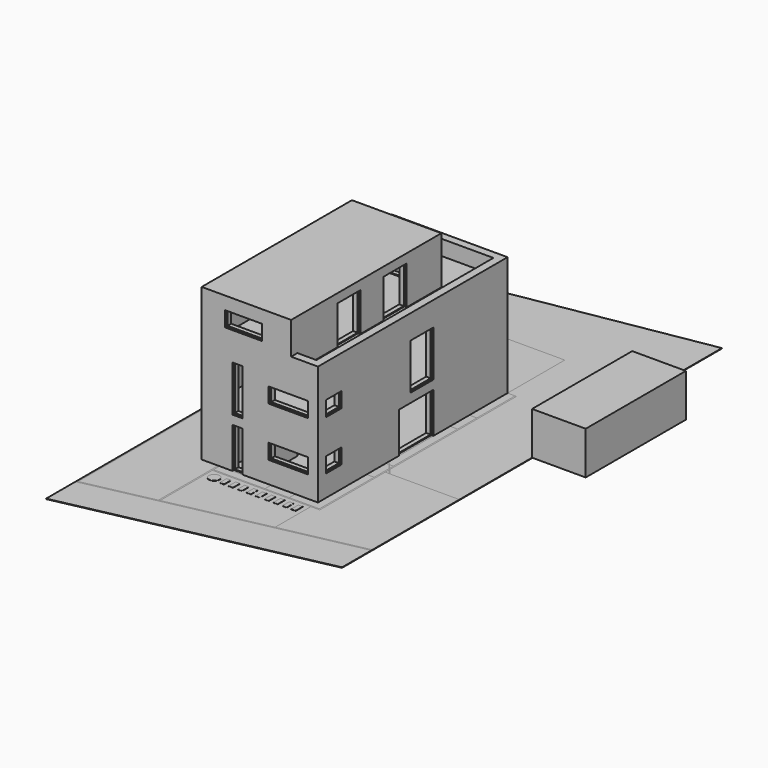
from build123d import *

# Parameters (mm, degrees)
F0_W      = 6500
F0_H      = 13250
F2_DEPTH  = 25
F3_DEPTH  = 2270
F1_W      = 150
F1_H      = 3500
F5_W      = 365
F5_H      = 1100
F5_W_2    = 2200
F5_H_2    = 365
F5_H_3    = 500
F6_DEPTH  = 850
F7_W      = 6500
F7_H      = 13250
F7_W_2    = 990
F7_H_2    = 2385
F8_DEPTH  = 300
F9_W      = 150
F9_H      = 3500
F10_DEPTH = 300
F11_W     = 6500
F11_H     = 13250
F12_DEPTH = 200
F14_DEPTH = 2570
F16_W     = 2200
F16_H     = 365
F16_W_2   = 365
F16_H_2   = 1100
F17_DEPTH = 850
F18_W     = 6500
F18_H     = 13250
F18_W_2   = 5770
F18_H_2   = 12520
F19_DEPTH = 300
F21_W     = 2400
F21_H     = 365
F22_DEPTH = 1280
F23_W     = 6500
F23_H     = 13250
F24_DEPTH = 200
F25_W     = 365
F25_H     = 1630
F26_DEPTH = 2160
F28_W     = 2050
F28_H     = 365
F29_DEPTH = 850
F30_W     = 5000
F30_H     = 10500
F30_W_2   = 4270
F30_H_2   = 9770
F31_DEPTH = 300
F32_W     = 5000
F32_H     = 10500
F33_DEPTH = 200
F35_DEPTH = 850
F38_DEPTH = 2200
F39_W     = 3000
F39_H     = 6000
F40_DEPTH = 25
F41_W     = 3000
F41_H     = 6000
F42_DEPTH = 200
F44_DEPTH = 25
F46_DEPTH = 25
F47_W     = 2880
F47_H     = 420
F48_DEPTH = 25
F47_W_2   = 420
F47_H_2   = 2670
F47_H_3   = 4480
F50_DEPTH = 25
F51_W     = 1350
F51_H     = 420
F52_DEPTH = 25
F51_W_2   = 420
F51_H_2   = 1350
F54_DEPTH = 25
F56_DEPTH = 25
F58_DEPTH = 25
F60_DEPTH = 25
F61_W     = 3000
F61_H     = 7000
F62_DEPTH = 2400
F63_R     = 1525
F64_DEPTH = 200
F65_R     = 1525
F65_R_2   = 1515
F66_DEPTH = 1800
F68_DEPTH = 25
F69_R     = 300
F70_DEPTH = 10
F71_W     = 250
F71_H     = 500
F72_DEPTH = 10
F74_DEPTH = 25
F76_DEPTH = 25
F77_W     = 570
F77_H     = 2570
F77_W_2   = 470
F77_H_2   = 2470
F78_DEPTH = 250
F77_W_3   = 2200
F77_H_3   = 850
F77_W_4   = 2100
F77_H_4   = 750
F77_W_5   = 2050
F77_W_6   = 1950
F77_H_5   = 2270
F77_H_6   = 2170
F79_W     = 2400
F79_H     = 2270
F79_W_2   = 2300
F79_H_2   = 2170
F80_DEPTH = 250
F79_W_3   = 1100
F79_H_3   = 850
F79_W_4   = 1000
F79_H_4   = 750
F79_W_5   = 1600
F79_H_5   = 2570
F79_W_6   = 1500
F79_H_6   = 2470
F81_W     = 1600
F81_H     = 2160
F81_W_2   = 1500
F81_H_2   = 2060
F82_DEPTH = 250
F83_W     = 2400
F83_H     = 1280
F83_W_2   = 2300
F83_H_2   = 1180
F84_DEPTH = 250
F83_H_3   = 2270
F83_H_4   = 2170
F85_W     = 2400
F85_H     = 2160
F85_W_2   = 2300
F85_H_2   = 2060
F86_DEPTH = 250
F87_W     = 570
F87_H     = 2570
F87_W_2   = 470
F87_H_2   = 2470
F88_DEPTH = 250
F87_W_3   = 1100
F87_H_3   = 2270
F87_W_4   = 1000
F87_H_4   = 2170
F87_W_5   = 500
F87_H_5   = 850
F87_W_6   = 400
F87_H_6   = 750
F89_W     = 2700
F89_H     = 2200
F90_DEPTH = 25
F91_W     = 850
F91_H     = 2200
F92_DEPTH = 25


with BuildPart() as f2:
    # F0 (on Top) → F2 (new body)
    with BuildSketch(Plane.XY):
        with Locations((3250, 6625)):
            Rectangle(F0_W, F0_H)
    extrude(amount=-F2_DEPTH)


with BuildPart() as f3:
    # F1 (on Top) → F3 (new body)
    with BuildSketch(Plane.XY):
        Polygon((2050, 12885), (2050, 13250), (0, 13250), (0, 4000), (365, 4000), (365, 12885), align=None)
    extrude(amount=F3_DEPTH)



with BuildPart() as f3b:
    # F1 (on Top) → F3, piece 2 (new body)
    with BuildSketch(Plane.XY):
        Polygon((4450, 13250), (4450, 12885), (6135, 12885), (6135, 8065), (6500, 8065), (6500, 13250), align=None)
    extrude(amount=F3_DEPTH)


with BuildPart() as f3c:
    # F1 (on Top) → F3, piece 3 (new body)
    with BuildSketch(Plane.XY):
        Polygon((6500, 5665), (6135, 5665), (6135, 1655), (6135, 555), (6135, 365), (5945, 365), (3745, 365), (3055, 365), (2955, 365), (2280, 365), (2280, 0), (3745, 0), (5945, 0), (6500, 0), (6500, 555), (6500, 1655), align=None)
        Polygon((2955, 365), (3055, 365), (3055, 2860), (2455, 2860), (2455, 2760), (2955, 2760), align=None)
    extrude(amount=F3_DEPTH)


with BuildPart() as f3d:
    # F1 (on Top) → F3, piece 4 (new body)
    with BuildSketch(Plane.XY):
        Polygon((1710, 0), (1710, 365), (1455, 365), (1355, 365), (365, 365), (365, 1400), (365, 1900), (365, 2750), (365, 2900), (0, 2900), (0, 1900), (0, 1400), (0, 0), align=None)
        Polygon((1355, 365), (1455, 365), (1455, 2900), (365, 2900), (365, 2750), (1355, 2750), align=None)
    extrude(amount=F3_DEPTH)


with BuildPart() as f3e:
    # F1 (on Top) → F3, piece 5 (new body)
    with BuildSketch(Plane.XY):
        with Locations((1380, 6250)):
            Rectangle(F1_W, F1_H)
    extrude(amount=F3_DEPTH)

    # F9 (on face) → F10 (join)
    with BuildSketch(Plane.XY.offset(2270)):
        with Locations((1380, 6250)):
            Rectangle(F9_W, F9_H)
    extrude(amount=F10_DEPTH)


with BuildPart() as f6_tool:
    # F5 (on offset) → F6 (new body)
    with BuildSketch(Plane.XY.offset(1200)):
        with Locations((6317.5, 1105)):
            Rectangle(F5_W, F5_H)
        with Locations((4845, 182.5)):
            Rectangle(F5_W_2, F5_H_2)
        with Locations((182.5, 1650)):
            Rectangle(F5_W, F5_H_3)
    extrude(amount=F6_DEPTH)


with BuildPart() as f3c_1:
    add(f3c.part)

    # F6: cut by f6_tool
    add(f6_tool.part, mode=Mode.SUBTRACT)


with BuildPart() as f3d_1:
    add(f3d.part)

    # F6: cut by f6_tool
    add(f6_tool.part, mode=Mode.SUBTRACT)


with BuildPart() as f3_1:
    add(f3.part)

    add(f3b.part)  # F8 merges F3b

    add(f3c_1.part)  # F8 merges F3c

    add(f3d_1.part)  # F8 merges F3d
    # F7 (on face) → F8 (join)
    with BuildSketch(Plane.XY.offset(2270)):
        with Locations((3250, 6625)):
            Rectangle(F7_W, F7_H)
        with Locations((860, 1557.5)):
            Rectangle(F7_W_2, F7_H_2, mode=Mode.SUBTRACT)
        Polygon((365, 2900), (365, 12885), (6135, 12885), (6135, 365), (3055, 365), (3055, 2860), (2455, 2860), (2455, 2760), (2955, 2760), (2955, 365), (1455, 365), (1455, 2900), align=None, mode=Mode.SUBTRACT)
    extrude(amount=F8_DEPTH)


    add(f3e.part)  # F12 merges F3e
    # F11 (on face) → F12 (join)
    with BuildSketch(Plane.XY.offset(2570)):
        with Locations((3250, 6625)):
            Rectangle(F11_W, F11_H)
    extrude(amount=F12_DEPTH)

    # F13 (on face) → F14 (join)
    with BuildSketch(Plane.XY.offset(2770)):
        Polygon((2050, 13250), (0, 13250), (0, 4210), (365, 4210), (365, 12885), (2050, 12885), (4450, 12885), (6135, 12885), (6135, 8065), (6500, 8065), (6500, 13250), (4450, 13250), align=None)
        Polygon((0, 3640), (0, 0), (1710, 0), (1710, 365), (365, 365), (365, 3640), align=None)
        Polygon((6500, 6465), (6135, 6465), (6135, 365), (2280, 365), (2280, 0), (6500, 0), align=None)
    extrude(amount=F14_DEPTH)

    # F16 (on offset) → F17 (cut)
    with BuildSketch(Plane.XY.offset(3970)):
        with Locations((4845, 182.5)):
            Rectangle(F16_W, F16_H)
        with Locations((6317.5, 1105)):
            Rectangle(F16_W_2, F16_H_2)
    extrude(amount=F17_DEPTH, mode=Mode.SUBTRACT)

    # F18 (on face) → F19 (join)
    with BuildSketch(Plane.XY.offset(5340)):
        with Locations((3250, 6625)):
            Rectangle(F18_W, F18_H)
        with Locations((3250, 6625)):
            Rectangle(F18_W_2, F18_H_2, mode=Mode.SUBTRACT)
    extrude(amount=F19_DEPTH)

    # F21 (on offset) → F22 (cut)
    with BuildSketch(Plane.XY.offset(3540)):
        with Locations((3250, 13067.5)):
            Rectangle(F21_W, F21_H)
    extrude(amount=F22_DEPTH, mode=Mode.SUBTRACT)

    # F23 (on face) → F24 (join)
    with BuildSketch(Plane.XY.offset(5640)):
        with Locations((3250, 6625)):
            Rectangle(F23_W, F23_H)
    extrude(amount=F24_DEPTH)

    # F25 (on face) → F26 (join)
    with BuildSketch(Plane.XY.offset(5840)):
        Polygon((0, 10500), (0, 0), (1310, 0), (3360, 0), (5000, 0), (5000, 3235), (4635, 3235), (4635, 365), (3360, 365), (1310, 365), (365, 365), (365, 10135), (2045, 10135), (2045, 10500), align=None)
        Polygon((4445, 10135), (4635, 10135), (4635, 8065), (5000, 8065), (5000, 10500), (4445, 10500), align=None)
        with Locations((4817.5, 5650)):
            Rectangle(F25_W, F25_H)
    extrude(amount=F26_DEPTH)

    # F28 (on offset) → F29 (cut)
    with BuildSketch(Plane.XY.offset(6930)):
        with Locations((2335, 182.5)):
            Rectangle(F28_W, F28_H)
    extrude(amount=F29_DEPTH, mode=Mode.SUBTRACT)

    # F30 (on face) → F31 (join)
    with BuildSketch(Plane.XY.offset(8000)):
        with Locations((2500, 5250)):
            Rectangle(F30_W, F30_H)
        with Locations((2500, 5250)):
            Rectangle(F30_W_2, F30_H_2, mode=Mode.SUBTRACT)
    extrude(amount=F31_DEPTH)

    # F32 (on face) → F33 (join)
    with BuildSketch(Plane.XY.offset(8300)):
        with Locations((2500, 5250)):
            Rectangle(F32_W, F32_H)
    extrude(amount=F33_DEPTH)

    # F34 (on face) → F35 (join)
    with BuildSketch(Plane.XY.offset(5840)):
        Polygon((0, 10500), (440, 10500), (440, 12810), (6060, 12810), (6060, 440), (5000, 440), (5000, 0), (6500, 0), (6500, 13250), (0, 13250), align=None)
    extrude(amount=F35_DEPTH)

    # F37 (on Top) → F38, piece 2 (join)
    with BuildSketch(Plane.XY):
        Polygon((-150, 6250), (0, 6250), (0, 12250), (-1750, 12250), (-1750, 12100), (-150, 12100), align=None)
    extrude(amount=F38_DEPTH)



with BuildPart() as f38:
    # F37 (on Top) → F38 (new body)
    with BuildSketch(Plane.XY):
        Polygon((-3000, 6250), (-2850, 6250), (-2850, 12100), (-2600, 12100), (-2600, 12250), (-3000, 12250), align=None)
    extrude(amount=F38_DEPTH)


with BuildPart() as f3_2:
    add(f3_1.part)

    add(f38.part)  # F40 merges F38
    # F39 (on Top) → F40 (join)
    with BuildSketch(Plane.XY):
        with Locations((-1500, 9250)):
            Rectangle(F39_W, F39_H)
    extrude(amount=-F40_DEPTH)

    # F41 (on face) → F42 (join)
    with BuildSketch(Plane.XY.offset(2200)):
        with Locations((-1500, 9250)):
            Rectangle(F41_W, F41_H)
    extrude(amount=F42_DEPTH)


with BuildPart() as f44:
    # F43 (on Top) → F44 (new body)
    with BuildSketch(Plane.XY):
        Polygon((-2920, 6250), (-3000, 6250), (-3000, -5000), (-2920, -4983.038869258), align=None)
    extrude(amount=-F44_DEPTH)


with BuildPart() as f44b:
    # F43 (on Top) → F44, piece 2 (new body)
    with BuildSketch(Plane.XY):
        Polygon((1000, 0), (920, 0), (920, -4168.9045936396), (1000, -4151.9434628975), align=None)
    extrude(amount=-F44_DEPTH)


with BuildPart() as f46:
    # F45 (on Top) → F46 (new body)
    with BuildSketch(Plane.XY):
        Polygon((-2920, 6250), (-2920, -4983.038869258), (920, -4168.9045936396), (920, 0), (0, 0), (0, 6250), align=None)
    extrude(amount=-F46_DEPTH)


with BuildPart() as f48:
    # F47 (on Top) → F48 (new body)
    with BuildSketch(Plane.XY):
        with Locations((2440, -210)):
            Rectangle(F47_W, F47_H)
    extrude(amount=-F48_DEPTH)


with BuildPart() as f48b:
    # F47 (on Top) → F48, piece 2 (new body)
    with BuildSketch(Plane.XY):
        Polygon((5230, -420), (6920, -420), (6920, 3400), (6500, 3400), (6500, 0), (5230, 0), align=None)
    extrude(amount=-F48_DEPTH)


with BuildPart() as f48c:
    # F47 (on Top) → F48, piece 3 (new body)
    with BuildSketch(Plane.XY):
        with Locations((6710, 11915)):
            Rectangle(F47_W_2, F47_H_2)
    extrude(amount=-F48_DEPTH)


with BuildPart() as f48d:
    # F47 (on Top) → F48, piece 4 (new body)
    with BuildSketch(Plane.XY):
        with Locations((6710, 6990)):
            Rectangle(F47_W_2, F47_H_3)
    extrude(amount=-F48_DEPTH)


with BuildPart() as f50:
    # F49 (on Top) → F50 (new body)
    with BuildSketch(Plane.XY):
        Polygon((1000, -420), (1000, -500), (7000, -500), (7000, 13250), (6920, 13250), (6920, -420), align=None)
    extrude(amount=-F50_DEPTH)


with BuildPart() as f52:
    # F51 (on Top) → F52 (new body)
    with BuildSketch(Plane.XY):
        with Locations((4555, -210)):
            Rectangle(F51_W, F51_H)
    extrude(amount=-F52_DEPTH)


with BuildPart() as f52b:
    # F51 (on Top) → F52, piece 2 (new body)
    with BuildSketch(Plane.XY):
        with Locations((6710, 4075)):
            Rectangle(F51_W_2, F51_H_2)
    extrude(amount=-F52_DEPTH)


with BuildPart() as f52c:
    # F51 (on Top) → F52, piece 3 (new body)
    with BuildSketch(Plane.XY):
        with Locations((6710, 9905)):
            Rectangle(F51_W_2, F51_H_2)
    extrude(amount=-F52_DEPTH)


with BuildPart() as f54:
    # F53 (on Top) → F54 (new body)
    with BuildSketch(Plane.XY):
        Polygon((1000, -500), (1000, -4151.9434628975), (6500, -2985.8657243816), (6500, -500), align=None)
    extrude(amount=-F54_DEPTH)


with BuildPart() as f56:
    # F55 (on Top) → F56 (new body)
    with BuildSketch(Plane.XY):
        Polygon((6500, -500), (6500, -2985.8657243816), (11150, -2000), (11150, 4075), (7000, 4075), (7000, -500), align=None)
    extrude(amount=-F56_DEPTH)


with BuildPart() as f58:
    # F57 (on Top) → F58 (new body)
    with BuildSketch(Plane.XY):
        Polygon((0, 14750), (0, 13250), (6500, 13250), (6500, 17250), (1500, 17250), (1500, 14750), align=None)
    extrude(amount=-F58_DEPTH)


with BuildPart() as f60:
    # F59 (on Top) → F60 (new body)
    with BuildSketch(Plane.XY):
        Polygon((11150, 22420), (-3000, 20000), (-3000, 12250), (0, 12250), (0, 14750), (1500, 14750), (1500, 17250), (6500, 17250), (6500, 13250), (7000, 13250), (7000, 4075), (11150, 4075), align=None)
    extrude(amount=-F60_DEPTH)


with BuildPart() as f62:
    # F61 (on Top) → F62 (new body)
    with BuildSketch(Plane.XY):
        with Locations((12650, 12650)):
            Rectangle(F61_W, F61_H)
    extrude(amount=F62_DEPTH)


with BuildPart() as f64:
    # F63 (on Top) → F64 (new body)
    with BuildSketch(Plane.XY):
        with Locations((-982.1203947067, 17554.7714233398)):
            Circle(F63_R)
    extrude(amount=F64_DEPTH)


with BuildPart() as f66:
    # F65 (on face) → F66 (new body)
    with BuildSketch(Plane.XY.offset(200)):
        with Locations((-982.1203947067, 17554.7714233398)):
            Circle(F65_R)
        with Locations((-982.1203947067, 17554.7714233398)):
            Circle(F65_R_2, mode=Mode.SUBTRACT)
    extrude(amount=F66_DEPTH)


with BuildPart() as f68:
    # F67 (on Top) → F68 (new body)
    with BuildSketch(Plane.XY):
        Polygon((6596.4529340073, 4828.9430343113), (7199.4075775146, 4094.8138237), (7230.1364810603, 4120.4211368522), (6621.9782528944, 4850.2140449441), align=None)
    extrude(amount=-F68_DEPTH)


with BuildPart() as f70:
    # F69 (on Top) → F70 (new body)
    with BuildSketch(Plane.XY):
        with Locations((1500, -1000)):
            Circle(F69_R)
    extrude(amount=F70_DEPTH)


with BuildPart() as f72:
    # F71 (on face) → F72 (new body)
    with BuildSketch(Plane.XY.offset(10)):
        with Locations((6125, -1000)):
            Rectangle(F71_W, F71_H)
    extrude(amount=F72_DEPTH)


with BuildPart() as f72b:
    # F71 (on face) → F72, piece 2 (new body)
    with BuildSketch(Plane.XY.offset(10)):
        with Locations((5625, -1000)):
            Rectangle(F71_W, F71_H)
    extrude(amount=F72_DEPTH)


with BuildPart() as f72c:
    # F71 (on face) → F72, piece 3 (new body)
    with BuildSketch(Plane.XY.offset(10)):
        with Locations((5125, -1000)):
            Rectangle(F71_W, F71_H)
    extrude(amount=F72_DEPTH)


with BuildPart() as f72d:
    # F71 (on face) → F72, piece 4 (new body)
    with BuildSketch(Plane.XY.offset(10)):
        with Locations((4625, -1000)):
            Rectangle(F71_W, F71_H)
    extrude(amount=F72_DEPTH)


with BuildPart() as f72e:
    # F71 (on face) → F72, piece 5 (new body)
    with BuildSketch(Plane.XY.offset(10)):
        with Locations((4125, -1000)):
            Rectangle(F71_W, F71_H)
    extrude(amount=F72_DEPTH)


with BuildPart() as f72f:
    # F71 (on face) → F72, piece 6 (new body)
    with BuildSketch(Plane.XY.offset(10)):
        with Locations((3625, -1000)):
            Rectangle(F71_W, F71_H)
    extrude(amount=F72_DEPTH)


with BuildPart() as f72g:
    # F71 (on face) → F72, piece 7 (new body)
    with BuildSketch(Plane.XY.offset(10)):
        with Locations((3125, -1000)):
            Rectangle(F71_W, F71_H)
    extrude(amount=F72_DEPTH)


with BuildPart() as f72h:
    # F71 (on face) → F72, piece 8 (new body)
    with BuildSketch(Plane.XY.offset(10)):
        with Locations((2625, -1000)):
            Rectangle(F71_W, F71_H)
    extrude(amount=F72_DEPTH)


with BuildPart() as f72i:
    # F71 (on face) → F72, piece 9 (new body)
    with BuildSketch(Plane.XY.offset(10)):
        with Locations((2125, -1000)):
            Rectangle(F71_W, F71_H)
    extrude(amount=F72_DEPTH)


with BuildPart() as f74:
    # F73 (on Top) → F74 (new body)
    with BuildSketch(Plane.XY):
        Polygon((11150, -2000), (-3000, -5000), (-3000, -5081.778236445), (11150, -2081.778236445), align=None)
    extrude(amount=-F74_DEPTH)


with BuildPart() as f76:
    # F75 (on Top) → F76 (new body)
    with BuildSketch(Plane.XY):
        Polygon((11150, -2081.778236445), (-3000, -5081.778236445), (-3000, -7126.2341475691), (11150, -4126.2341475691), align=None)
    extrude(amount=-F76_DEPTH)


with BuildPart() as f78:
    # F77 (on face) → F78 (new body)
    with BuildSketch(Plane(origin=(0, 365, 0), x_dir=(-1, 0, 0), z_dir=(0, 1, 0))):
        with Locations((-1995, 4055)):
            Rectangle(F77_W, F77_H)
        with Locations((-1995, 4055)):
            Rectangle(F77_W_2, F77_H_2, mode=Mode.SUBTRACT)
    extrude(amount=-F78_DEPTH)


with BuildPart() as f78b:
    # F77 (on face) → F78, piece 2 (new body)
    with BuildSketch(Plane(origin=(0, 365, 0), x_dir=(-1, 0, 0), z_dir=(0, 1, 0))):
        with Locations((-4845, 4395)):
            Rectangle(F77_W_3, F77_H_3)
        with Locations((-4845, 4395)):
            Rectangle(F77_W_4, F77_H_4, mode=Mode.SUBTRACT)
    extrude(amount=-F78_DEPTH)


with BuildPart() as f78c:
    # F77 (on face) → F78, piece 3 (new body)
    with BuildSketch(Plane(origin=(0, 365, 0), x_dir=(-1, 0, 0), z_dir=(0, 1, 0))):
        with Locations((-2335, 7355)):
            Rectangle(F77_W_5, F77_H_3)
        with Locations((-2335, 7355)):
            Rectangle(F77_W_6, F77_H_4, mode=Mode.SUBTRACT)
    extrude(amount=-F78_DEPTH)


with BuildPart() as f78d:
    # F77 (on face) → F78, piece 4 (new body)
    with BuildSketch(Plane(origin=(0, 365, 0), x_dir=(-1, 0, 0), z_dir=(0, 1, 0))):
        with Locations((-1995, 1135)):
            Rectangle(F77_W, F77_H_5)
        with Locations((-1995, 1135)):
            Rectangle(F77_W_2, F77_H_6, mode=Mode.SUBTRACT)
    extrude(amount=-F78_DEPTH)


with BuildPart() as f78e:
    # F77 (on face) → F78, piece 5 (new body)
    with BuildSketch(Plane(origin=(0, 365, 0), x_dir=(-1, 0, 0), z_dir=(0, 1, 0))):
        with Locations((-4845, 1625)):
            Rectangle(F77_W_3, F77_H_3)
        with Locations((-4845, 1625)):
            Rectangle(F77_W_4, F77_H_4, mode=Mode.SUBTRACT)
    extrude(amount=-F78_DEPTH)


with BuildPart() as f80:
    # F79 (on face) → F80 (new body)
    with BuildSketch(Plane(origin=(6135, 0, 0), x_dir=(0, -1, 0), z_dir=(-1, 0, 0))):
        with Locations((-6865, 1135)):
            Rectangle(F79_W, F79_H)
        with Locations((-6865, 1135)):
            Rectangle(F79_W_2, F79_H_2, mode=Mode.SUBTRACT)
    extrude(amount=-F80_DEPTH)


with BuildPart() as f80b:
    # F79 (on face) → F80, piece 2 (new body)
    with BuildSketch(Plane(origin=(6135, 0, 0), x_dir=(0, -1, 0), z_dir=(-1, 0, 0))):
        with Locations((-1105, 1625)):
            Rectangle(F79_W_3, F79_H_3)
        with Locations((-1105, 1625)):
            Rectangle(F79_W_4, F79_H_4, mode=Mode.SUBTRACT)
    extrude(amount=-F80_DEPTH)


with BuildPart() as f80c:
    # F79 (on face) → F80, piece 3 (new body)
    with BuildSketch(Plane(origin=(6135, 0, 0), x_dir=(0, -1, 0), z_dir=(-1, 0, 0))):
        with Locations((-1105, 4395)):
            Rectangle(F79_W_3, F79_H_3)
        with Locations((-1105, 4395)):
            Rectangle(F79_W_4, F79_H_4, mode=Mode.SUBTRACT)
    extrude(amount=-F80_DEPTH)


with BuildPart() as f80d:
    # F79 (on face) → F80, piece 4 (new body)
    with BuildSketch(Plane(origin=(6135, 0, 0), x_dir=(0, -1, 0), z_dir=(-1, 0, 0))):
        with Locations((-7265, 4055)):
            Rectangle(F79_W_5, F79_H_5)
        with Locations((-7265, 4055)):
            Rectangle(F79_W_6, F79_H_6, mode=Mode.SUBTRACT)
    extrude(amount=-F80_DEPTH)


with BuildPart() as f82:
    # F81 (on face) → F82 (new body)
    with BuildSketch(Plane(origin=(4635, 0, 0), x_dir=(0, -1, 0), z_dir=(-1, 0, 0))):
        with Locations((-4035, 6920)):
            Rectangle(F81_W, F81_H)
        with Locations((-4035, 6920)):
            Rectangle(F81_W_2, F81_H_2, mode=Mode.SUBTRACT)
    extrude(amount=-F82_DEPTH)


with BuildPart() as f82b:
    # F81 (on face) → F82, piece 2 (new body)
    with BuildSketch(Plane(origin=(4635, 0, 0), x_dir=(0, -1, 0), z_dir=(-1, 0, 0))):
        with Locations((-7265, 6920)):
            Rectangle(F81_W, F81_H)
        with Locations((-7265, 6920)):
            Rectangle(F81_W_2, F81_H_2, mode=Mode.SUBTRACT)
    extrude(amount=-F82_DEPTH)


with BuildPart() as f84:
    # F83 (on face) → F84 (new body)
    with BuildSketch(Plane.XZ.offset(-12885)):
        with Locations((3250, 4180)):
            Rectangle(F83_W, F83_H)
        with Locations((3250, 4180)):
            Rectangle(F83_W_2, F83_H_2, mode=Mode.SUBTRACT)
    extrude(amount=-F84_DEPTH)


with BuildPart() as f84b:
    # F83 (on face) → F84, piece 2 (new body)
    with BuildSketch(Plane.XZ.offset(-12885)):
        with Locations((3250, 1135)):
            Rectangle(F83_W, F83_H_3)
        with Locations((3250, 1135)):
            Rectangle(F83_W_2, F83_H_4, mode=Mode.SUBTRACT)
    extrude(amount=-F84_DEPTH)


with BuildPart() as f86:
    # F85 (on face) → F86 (new body)
    with BuildSketch(Plane.XZ.offset(-10135)):
        with Locations((3245, 6920)):
            Rectangle(F85_W, F85_H)
        with Locations((3245, 6920)):
            Rectangle(F85_W_2, F85_H_2, mode=Mode.SUBTRACT)
    extrude(amount=-F86_DEPTH)


with BuildPart() as f88:
    # F87 (on face) → F88 (new body)
    with BuildSketch(Plane.YZ.offset(365)):
        with Locations((3925, 4055)):
            Rectangle(F87_W, F87_H)
        with Locations((3925, 4055)):
            Rectangle(F87_W_2, F87_H_2, mode=Mode.SUBTRACT)
    extrude(amount=-F88_DEPTH)


with BuildPart() as f88b:
    # F87 (on face) → F88, piece 2 (new body)
    with BuildSketch(Plane.YZ.offset(365)):
        with Locations((3450, 1135)):
            Rectangle(F87_W_3, F87_H_3)
        with Locations((3450, 1135)):
            Rectangle(F87_W_4, F87_H_4, mode=Mode.SUBTRACT)
    extrude(amount=-F88_DEPTH)


with BuildPart() as f88c:
    # F87 (on face) → F88, piece 3 (new body)
    with BuildSketch(Plane.YZ.offset(365)):
        with Locations((1650, 1625)):
            Rectangle(F87_W_5, F87_H_5)
        with Locations((1650, 1625)):
            Rectangle(F87_W_6, F87_H_6, mode=Mode.SUBTRACT)
    extrude(amount=-F88_DEPTH)


with BuildPart() as f90:
    # F89 (on face) → F90 (new body)
    with BuildSketch(Plane.XZ.offset(-6250)):
        with Locations((-1500, 1100)):
            Rectangle(F89_W, F89_H)
    extrude(amount=-F90_DEPTH)


with BuildPart() as f92:
    # F91 (on face) → F92 (new body)
    with BuildSketch(Plane(origin=(0, 12250, 0), x_dir=(-1, 0, 0), z_dir=(0, 1, 0))):
        with Locations((2175, 1100)):
            Rectangle(F91_W, F91_H)
    extrude(amount=-F92_DEPTH)


solid = Compound([f2.part, f3_2.part, f44.part, f44b.part, f46.part, f48.part, f48b.part, f48c.part, f48d.part, f50.part, f52.part, f52b.part, f52c.part, f54.part, f56.part, f58.part, f60.part, f62.part, f64.part, f66.part, f68.part, f70.part, f72.part, f72b.part, f72c.part, f72d.part, f72e.part, f72f.part, f72g.part, f72h.part, f72i.part, f74.part, f76.part, f78.part, f78b.part, f78c.part, f78d.part, f78e.part, f80.part, f80b.part, f80c.part, f80d.part, f82.part, f82b.part, f84.part, f84b.part, f86.part, f88.part, f88b.part, f88c.part, f90.part, f92.part])
